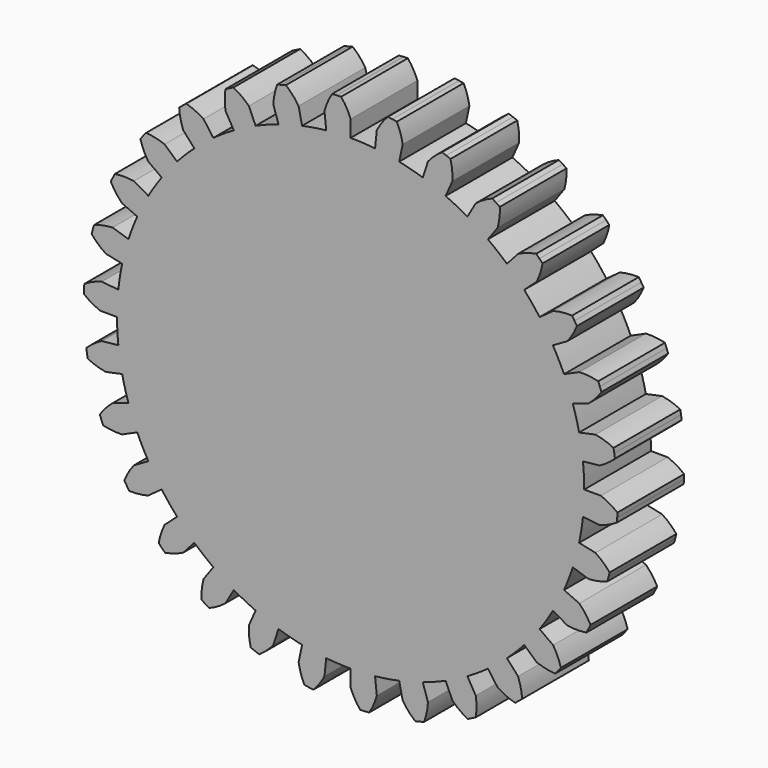
from build123d import *

# Parameters (mm, degrees)
F2_DEPTH        = 10
F2_COPIES_COUNT = 30


# Not quite as in the source:
# - a feature of the source that left no trace in its solid (it failed there, or was rolled back) is left out
# - a pattern or mirror of a feature is missing from the dataset's text; its kind, count and spacing are read off the source's solid


with BuildPart() as f2:
    # F1 (on Front) → F2 (new body, symmetric)
    with BuildSketch(Plane.XZ):
        with BuildLine():
            ThreePointArc((-5.853593943, 55.6932261406), (-37.4713139561, -41.6161102267), (56, 0))
            ThreePointArc((56, 0), (39.5979797464, 39.5979797464), (0, 56))
            ThreePointArc((0, 56), (-2.9308135496, 55.9232539463), (-5.853593943, 55.6932261406))
        make_face()
        with BuildLine():
            ThreePointArc((-5.853593943, 55.6932261406), (-2.9308135496, 55.9232539463), (0, 56))
            Line((0, 56), (0, 60))
            ThreePointArc((0, 60), (-0.9817353122, 62.066603372), (-2.2663496541, 63.95985975))
            ThreePointArc((-2.2663496541, 63.95985975), (-2.8080261604, 63.938368677), (-3.3495011995, 63.9122902243))
            ThreePointArc((-3.3495011995, 63.9122902243), (-3.8907359223, 63.8816262628), (-4.4316914969, 63.8463789927))
            ThreePointArc((-4.4316914969, 63.8463789927), (-5.5113694073, 61.8292153081), (-6.2717077961, 59.6713137221))
            Line((-6.2717077961, 59.6713137221), (-5.853593943, 55.6932261406))
        make_face()
    extrude(amount=F2_DEPTH, both=True)

    # F2_copies: F2 ×30 about axis
    f2_copies_axis = Axis((0, 0, 0), (0, 1, 0))


with BuildPart() as f2_1:
    add(f2.part)
    for i in range(1, F2_COPIES_COUNT):
        add(f2.part.rotate(f2_copies_axis, i * 360 / F2_COPIES_COUNT))


solid = f2_1.part
